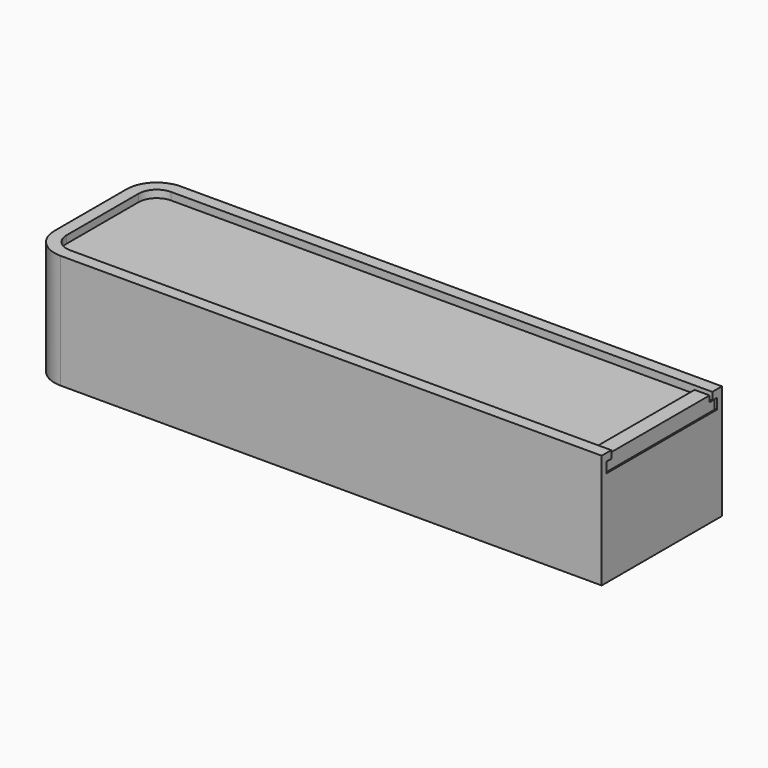
from build123d import *

# Parameters (mm, degrees)
F1_DEPTH  = 38
F2_DEPTH  = 4
F3_W      = 42
F3_H      = 2.5
F4_DEPTH  = 180
F5_W      = 2
F5_H      = 3.5
F8_DEPTH  = 3
F9_W      = 5
F9_H      = 41
F10_DEPTH = 2


# Not quite as in the source:
# - a feature names something its author has since deleted; it is built from what else it names


with BuildPart() as f1:
    # F0 (on Top) → F1 (new body)
    with BuildSketch(Plane.XY):
        with BuildLine():
            ThreePointArc((-91, 15), (-89.2426406871, 19.2426406871), (-85, 21))
            Line((-85, 21), (-85, 25))
            ThreePointArc((-85, 25), (-92.0710678119, 22.0710678119), (-95, 15))
            Line((-95, 15), (-91, 15))
        make_face()
        with BuildLine():
            Line((91, 21), (91, -21))
            Line((91, -21), (-85, -21))
            ThreePointArc((-85, -21), (-89.2426406871, -19.2426406871), (-91, -15))
            Line((-91, -15), (-91, 15))
            Line((-91, 15), (-95, 15))
            Line((-95, 15), (-95, -15))
            ThreePointArc((-95, -15), (-92.0710678119, -22.0710678119), (-85, -25))
            Line((-85, -25), (95, -25))
            Line((95, -25), (95, 25))
            Line((95, 25), (-85, 25))
            Line((-85, 25), (-85, 21))
            Line((-85, 21), (91, 21))
        make_face()
    extrude(amount=F1_DEPTH)

    # F0 (on Top) → F2 (join)
    with BuildSketch(Plane.XY):
        with BuildLine():
            Line((-85, -21), (91, -21))
            Line((91, -21), (91, 21))
            Line((91, 21), (-85, 21))
            ThreePointArc((-85, 21), (-89.2426406871, 19.2426406871), (-91, 15))
            Line((-91, 15), (-91, -15))
            ThreePointArc((-91, -15), (-89.2426406871, -19.2426406871), (-85, -21))
        make_face()
    extrude(amount=F2_DEPTH)

    # F3 (on face) → F4 (cut, through all)
    with BuildSketch(Plane.YZ.offset(95)):
        with Locations((0, 36.75)):
            Rectangle(F3_W, F3_H)
        Polygon((21, 35.5), (-21, 35.5), (-23, 35.5), (-23, 32), (-21, 32), (21, 32), (23, 32), (23, 35.5), align=None)
    extrude(amount=-F4_DEPTH, mode=Mode.SUBTRACT)

    # F6: sweep along a path in F6_path
    with BuildLine(Plane(origin=(-91, -15, 38), x_dir=(0, -1, 0), z_dir=(0, 0, -1))) as f6_path:
        ThreePointArc((6, -6), (4.2426406871, -1.7573593129), (0, 0))
        Line((0, 0), (-30, 0))
        ThreePointArc((-30, 0), (-34.2426406871, -1.7573593129), (-36, -6))
    # F5 (on face) → F6 (sweep, cut)
    with BuildSketch(Plane.YZ.offset(-85)):
        with Locations((-22, 33.75)):
            Rectangle(F5_W, F5_H)
    sweep(path=f6_path.line, mode=Mode.SUBTRACT)


with BuildPart() as f8:
    # F7 (on face) → F8 (new body)
    with BuildSketch(Plane.XY.offset(32)):
        with BuildLine():
            Line((94.4999977946, 22.4999977946), (-85, 22.4999977946))
            ThreePointArc((-85, 22.4999977946), (-90.3032992995, 20.3032992995), (-92.4999977946, 15))
            Line((-92.4999977946, 15), (-92.4999977946, -15))
            ThreePointArc((-92.4999977946, -15), (-90.3032992995, -20.3032992995), (-85, -22.4999977946))
            Line((-85, -22.4999977946), (94.4999977946, -22.4999977946))
            Line((94.4999977946, -22.4999977946), (94.4999977946, 22.4999977946))
        make_face()
        with BuildLine():
            ThreePointArc((-91, 15), (-89.2426406871, 19.2426406871), (-85, 21))
            Line((-85, 21), (91, 21))
            Line((91, 21), (91, -21))
            Line((91, -21), (-85, -21))
            ThreePointArc((-85, -21), (-89.2426406871, -19.2426406871), (-91, -15))
            Line((-91, -15), (-91, 15))
        make_face(mode=Mode.SUBTRACT)
        with BuildLine():
            Line((91, 21), (-85, 21))
            ThreePointArc((-85, 21), (-89.2426406871, 19.2426406871), (-91, 15))
            Line((-91, 15), (-91, -15))
            ThreePointArc((-91, -15), (-89.2426406871, -19.2426406871), (-85, -21))
            Line((-85, -21), (91, -21))
            Line((91, -21), (91, 21))
        make_face()
    extrude(amount=F8_DEPTH)

    # F9 (on face) → F10 (join, through all)
    with BuildSketch(Plane.XY.offset(35)):
        with Locations((91.9999977946, 0)):
            Rectangle(F9_W, F9_H)
    extrude(amount=F10_DEPTH)


solid = Compound([f1.part, f8.part])
